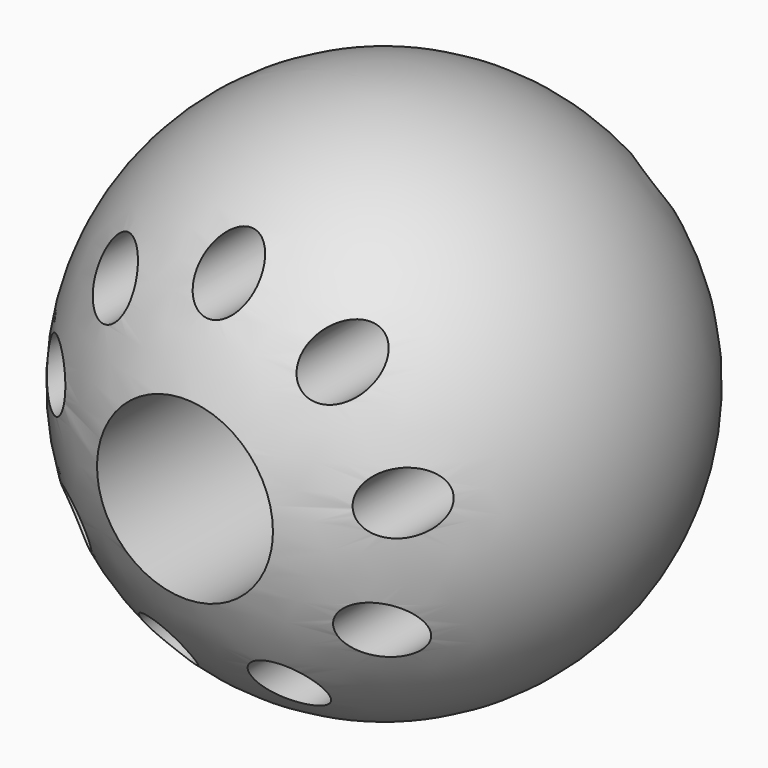
from build123d import *

# Parameters (mm, degrees)
F2_R     = 50
F2_R_2   = 16.66665
F3_DEPTH = 150


# Not quite as in the source:
# - a feature of the source that left no trace in its solid (it failed there, or was rolled back) is left out


with BuildPart() as f1:
    # F0 (on Front) → F1 (revolve)
    with BuildSketch(Plane.XZ):
        with BuildLine():
            Line((0, -150), (0, 150))
            ThreePointArc((0, 150), (-150, 0), (0, -150))
        make_face()
    revolve(axis=Axis((0, 0, -0.4973262548), (0, 0, -1)))

    # F2 (on Front) → F3 (cut, symmetric)
    with BuildSketch(Plane.XZ):
        Circle(F2_R)
        with Locations((0, 100)):
            Circle(F2_R_2)
        with Locations((-64.2787609687, 76.6044443119)):
            Circle(F2_R_2)
        with Locations((-98.4807753012, 17.3648177667)):
            Circle(F2_R_2)
        with Locations((-86.6025403784, -50)):
            Circle(F2_R_2)
        with Locations((-34.2020143326, -93.9692620786)):
            Circle(F2_R_2)
        with Locations((34.2020143326, -93.9692620786)):
            Circle(F2_R_2)
        with Locations((86.6025403784, -50)):
            Circle(F2_R_2)
        with Locations((98.4807753012, 17.3648177667)):
            Circle(F2_R_2)
        with Locations((64.2787609687, 76.6044443119)):
            Circle(F2_R_2)
    extrude(amount=F3_DEPTH, both=True, mode=Mode.SUBTRACT)


solid = f1.part
